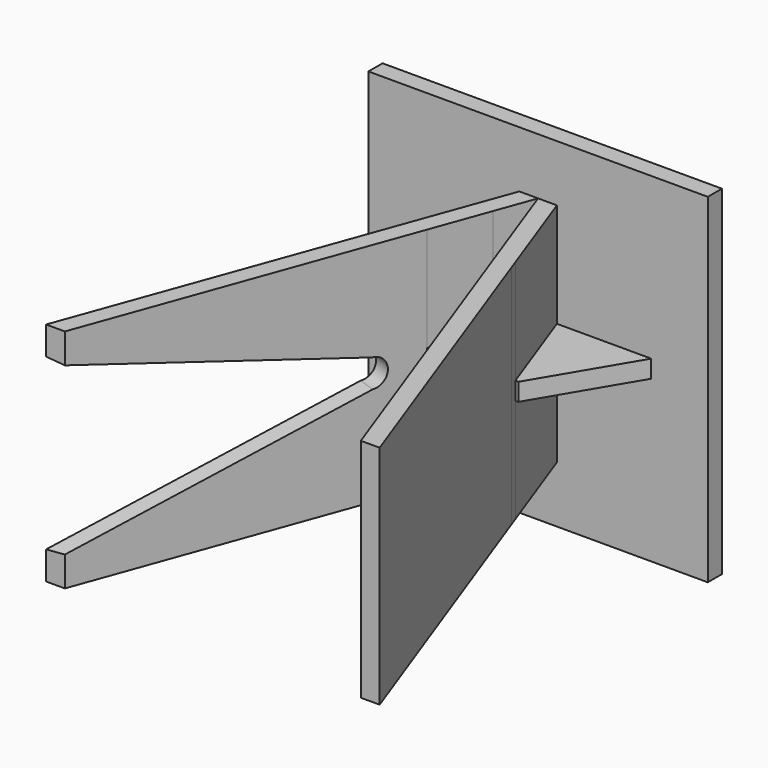
from build123d import *

# Parameters (mm, degrees)
F0_W          = 304.8
F0_H          = 304.8
F0_W_2        = 101.6
F0_H_2        = 15.875
F1_DEPTH      = 15.875
F3_DEPTH      = 7.9375
F3_DEPTH_BACK = 7.9375
F4_DEPTH      = 101.6
F4_DEPTH_BACK = 101.6
F5_DEPTH      = 7.9375
F5_DEPTH_BACK = 7.9375
F7_DEPTH      = 25.4


with BuildPart() as f1:
    # F0 (on Front) → F1 (new body)
    with BuildSketch(Plane.XZ):
        Rectangle(F0_W, F0_H)
        Rectangle(F0_W_2, F0_H_2, mode=Mode.SUBTRACT)
    extrude(amount=F1_DEPTH)


with BuildPart() as f3:
    # F2 (on Top) → F3 (new body, two sides)
    with BuildSketch(Plane.XY) as f3_sk:
        Polygon((-50.8, -50.8), (-50.8, -15.875), (-101.6, -15.875), (-50.8, -101.6), align=None)
        Polygon((50.8, 0), (-50.8, 0), (-50.8, -15.875), (-50.8, -50.8), (-29.6054825698, -50.8), (-16.8938221381, -15.875), (0, -15.875), (16.8938221381, -15.875), (29.6054825698, -50.8), (50.8, -50.8), (50.8, -15.875), align=None)
        Polygon((101.6, -15.875), (50.8, -15.875), (50.8, -50.8), (50.8, -101.6), align=None)
        Polygon((12.7116604317, -50.8), (-12.7116604317, -50.8), (-31.2013483325, -101.6), (31.2013483325, -101.6), align=None)
        Polygon((-16.8938221381, -15.875), (-29.6054825698, -50.8), (-12.7116604317, -50.8), (0, -15.875), align=None)
        Polygon((-29.6054825698, -50.8), (-50.8, -50.8), (-50.8, -101.6), (-48.0951704705, -101.6), align=None)
        Polygon((12.7116604317, -50.8), (29.6054825698, -50.8), (16.8938221381, -15.875), (0, -15.875), align=None)
        Polygon((50.8, -101.6), (50.8, -50.8), (29.6054825698, -50.8), (48.0951704705, -101.6), align=None)
        Polygon((0, -15.875), (-12.7116604317, -50.8), (12.7116604317, -50.8), align=None)
    extrude(amount=F3_DEPTH)
    extrude(f3_sk.sketch, amount=-F3_DEPTH_BACK)


with BuildPart() as f4:
    # F2 (on Top) → F4 (new body, two sides)
    with BuildSketch(Plane.XY) as f4_sk:
        Polygon((-16.8938221381, -15.875), (-29.6054825698, -50.8), (-12.7116604317, -50.8), (0, -15.875), align=None)
        Polygon((-31.2013483325, -101.6), (-48.0951704705, -101.6), (-50.8, -109.0314580557), (-149.7884539245, -381), (-132.8946317864, -381), align=None)
        Polygon((-12.7116604317, -50.8), (-29.6054825698, -50.8), (-48.0951704705, -101.6), (-31.2013483325, -101.6), align=None)
    extrude(amount=F4_DEPTH)
    extrude(f4_sk.sketch, amount=-F4_DEPTH_BACK)

    # F2 (on Top) → F5 (cut, two sides)
    with BuildSketch(Plane.XY) as f5_sk:
        Polygon((-16.8938221381, -15.875), (-29.6054825698, -50.8), (-12.7116604317, -50.8), (0, -15.875), align=None)
        Polygon((12.7116604317, -50.8), (29.6054825698, -50.8), (16.8938221381, -15.875), (0, -15.875), align=None)
    extrude(amount=F5_DEPTH, mode=Mode.SUBTRACT)
    extrude(f5_sk.sketch, amount=-F5_DEPTH_BACK, mode=Mode.SUBTRACT)

    # F6 (on face) → F7 (cut)
    with BuildSketch(Plane(origin=(-9.8154937031, 3.5725475426, 0), x_dir=(-0.3420201433, -0.9396926208, 0), z_dir=(-0.9396926208, 0.3420201433, 0))):
        with BuildLine():
            ThreePointArc((150.9473935528, 12.7), (159.9276496739, 8.9802561211), (163.6473935528, 0))
            ThreePointArc((163.6473935528, 0), (159.9276496739, -8.9802561211), (150.9473935528, -12.7))
            Line((150.9473935528, -12.7), (409.2535569992, -76.2))
            Line((409.2535569992, -76.2), (409.2535569992, 76.2))
            Line((409.2535569992, 76.2), (150.9473935528, 12.7))
        make_face()
        with BuildLine():
            ThreePointArc((150.9473935528, -12.7), (159.9276496739, -8.9802561211), (163.6473935528, 0))
            ThreePointArc((163.6473935528, 0), (159.9276496739, 8.9802561211), (150.9473935528, 12.7))
            ThreePointArc((150.9473935528, 12.7), (138.2473935528, 0), (150.9473935528, -12.7))
        make_face()
    extrude(amount=-F7_DEPTH, mode=Mode.SUBTRACT)


with BuildPart() as f4b:
    # F2 (on Top) → F4, piece 2 (new body, two sides)
    with BuildSketch(Plane.XY) as f4_2_sk:
        Polygon((12.7116604317, -50.8), (29.6054825698, -50.8), (16.8938221381, -15.875), (0, -15.875), align=None)
        Polygon((48.0951704705, -101.6), (29.6054825698, -50.8), (12.7116604317, -50.8), (31.2013483325, -101.6), align=None)
        Polygon((50.8, -109.0314580557), (48.0951704705, -101.6), (31.2013483325, -101.6), (132.8946317864, -381), (149.7884539245, -381), align=None)
    extrude(amount=F4_DEPTH)
    extrude(f4_2_sk.sketch, amount=-F4_DEPTH_BACK)


solid = Compound([f1.part, f3.part, f4.part, f4b.part])
